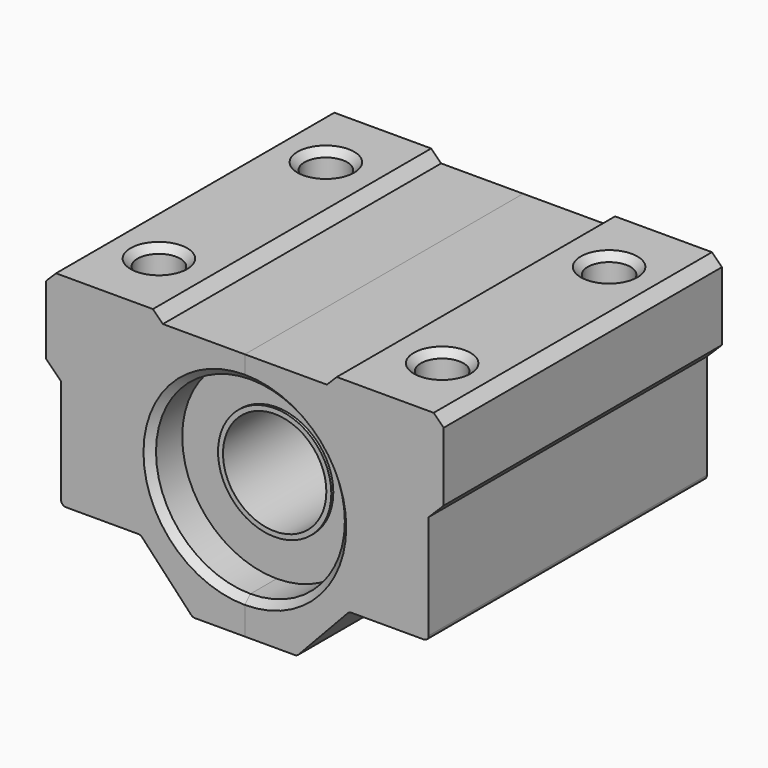
from build123d import *
from build123d import SkipClean  # not in build123d's __all__

# Parameters (mm, degrees)
F1_DEPTH       = 17.5
F2_SIZE        = 0.99999
F3_SIZE        = 1.49999
F4_R           = 0.5
F6_D           = 4
F6_CBORE_D     = 4.3
F6_CBORE_DEPTH = 12
F7_SIZE        = 0.7
F0_R           = 5.7
F8_DEPTH       = 13.5
F0_R_2         = 5.2
F9_DEPTH       = 13.75


# Not quite as in the source:
# - a fillet or chamfer is up to 0.001 mm smaller than in the source, because OpenCascade refuses the exact size


with BuildPart() as f1:
    # F0 (on Front) → F1 (new body, symmetric)
    with BuildSketch(Plane.XZ):
        with BuildLine():
            ThreePointArc((0, 9.5), (6.7175144213, 6.7175144213), (9.5, 0))
            ThreePointArc((9.5, 0), (6.7175144213, -6.7175144213), (0, -9.5))
            Line((0, -9.5), (0, -13))
            Line((0, -13), (5.25, -13))
            Line((5.25, -13), (10.5, -7.4))
            Line((10.5, -7.4), (18.5, -7.4))
            Line((18.5, -7.4), (18.5, 3.6))
            Line((18.5, 3.6), (20, 3.6))
            Line((20, 3.6), (20, 13))
            Line((20, 13), (9.25, 13))
            Line((9.25, 13), (9.25, 12))
            Line((9.25, 12), (0, 12))
            Line((0, 12), (0, 9.5))
        make_face()
    extrude(amount=F1_DEPTH, both=True)

    # F2 (size 1 in the source; OpenCascade refuses exactly that, so slightly less here)
    f2_edges = [f1.edges().sort_by_distance(p)[0] for p in [
        (9.25, 0, 12),
        (20, 0, 13),
    ]]
    chamfer(f2_edges, length=F2_SIZE)

    # F3 (size 1.5 in the source; OpenCascade refuses exactly that, so slightly less here)
    f3_edges = [f1.edges().sort_by_distance(p)[0] for p in [
        (20, 0, 3.6),
    ]]
    chamfer(f3_edges, length=F3_SIZE)

    # F4
    f4_edges = [f1.edges().sort_by_distance(p)[0] for p in [
        (18.5, 0, -7.4),
        (10.5, 0, -7.4),
        (5.25, 0, -13),
    ]]
    fillet(f4_edges, radius=F4_R)

    # F6 (through all)
    with Locations(Plane.XY.offset(13)):
        with Locations((14.25, 10.5), (14.25, -10.5)):
            CounterBoreHole(F6_D / 2, F6_CBORE_D / 2, F6_CBORE_DEPTH)

    # F7
    f7_edges = [f1.edges().sort_by_distance(p)[0] for p in [
        (9.5, -17.5, 0),
        (9.5, 17.5, 0),
        (12.1, 10.5, 13),
        (12.1, -10.5, 13),
    ]]
    chamfer(f7_edges, length=F7_SIZE)

    # F10: F1 across plane


with BuildPart() as f8:
    # F0 (on Front) → F8 (new body, symmetric)
    with BuildSketch(Plane.XZ):
        with BuildLine():
            ThreePointArc((0, -9.5), (6.7175144213, -6.7175144213), (9.5, 0))
            ThreePointArc((9.5, 0), (6.7175144213, 6.7175144213), (0, 9.5))
            ThreePointArc((0, 9.5), (-9.5, 0), (0, -9.5))
        make_face()
        Circle(F0_R, mode=Mode.SUBTRACT)
    extrude(amount=F8_DEPTH, both=True)

    # F0 (on Front) → F9 (join, symmetric)
    with BuildSketch(Plane.XZ):
        Circle(F0_R)
        Circle(F0_R_2, mode=Mode.SUBTRACT)
    extrude(amount=F9_DEPTH, both=True)


with BuildPart() as f1_1:
    add(f1.part, clean=False)
    with SkipClean():  # cleaning this boolean's faces spoils the solid; the shape is the same uncleaned
        add(f1.part.mirror(Plane.YZ), clean=False)


solid = Compound([f8.part, f1_1.part])
